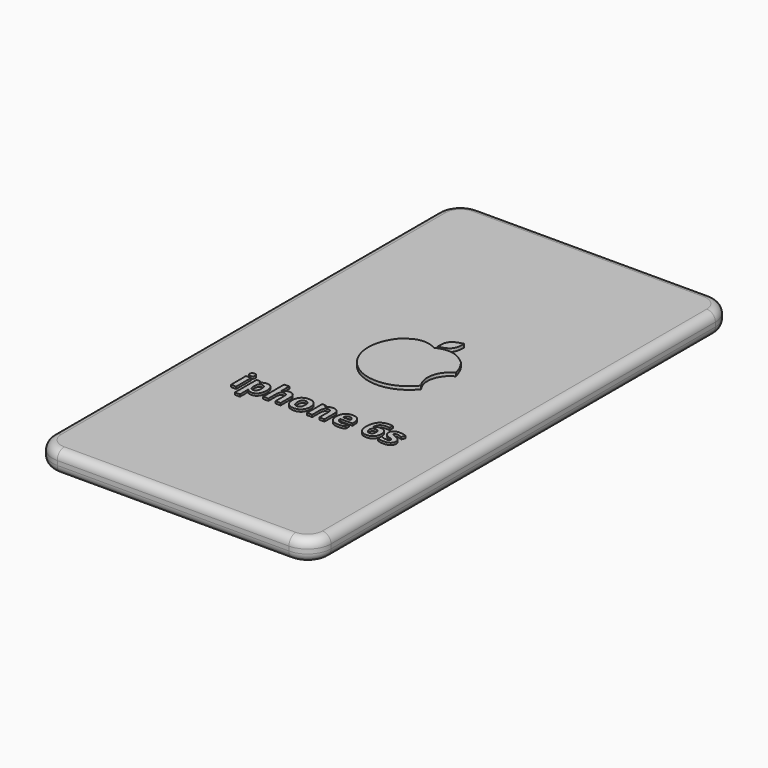
from build123d import *

# Parameters (mm, degrees)
F0_W         = 129.3353596702
F0_H         = 244.9735552073
F1_DEPTH     = 10
F3_W         = 97.1785942093
F3_H         = 200.6838843226
F3_R         = 8.9904805896
F4_DEPTH     = 1
F5_R         = 10.8639610307
F6_R         = 4
F7_TEXT_SIZE = 15.9748014994
F8_DEPTH     = 1
F10_DEPTH    = 1.5
F12_DEPTH    = 1.5


# Not quite as in the source:
# - Text() gives the source's letters only with a copy of the font that has no kerning and outlines rounded to 1/6400 em; it was checked with that copy


with BuildPart() as f1:
    # F0 (on Top) → F1 (new body)
    with BuildSketch(Plane.XY):
        with Locations((-4.1642035358, 44.1017150879)):
            Rectangle(F0_W, F0_H)
    extrude(amount=-F1_DEPTH)

    # F3 (on face) → F4 (cut)
    with BuildSketch(Plane(origin=(0, 0, -10), x_dir=(1, 0, 0), z_dir=(0, 0, -1))):
        with Locations((-4.1642035358, -38.0352623761)):
            Rectangle(F3_W, F3_H)
        with Locations((-11.1623336561, -151.3912901282)):
            Circle(F3_R)
        with BuildLine():
            ThreePointArc((-19.1459041089, 70.0142735839), (-20.1459041089, 69.0142735839), (-19.1459041089, 68.0142735839))
            Line((-19.1459041089, 68.0142735839), (0, 68.0142735839))
            ThreePointArc((0, 68.0142735839), (1, 69.0142735839), (0, 70.0142735839))
            Line((0, 70.0142735839), (-19.1459041089, 70.0142735839))
        make_face()
    extrude(amount=-F4_DEPTH, mode=Mode.SUBTRACT)

    # F5
    f5_edges = [f1.edges().sort_by_distance(p)[0] for p in [
        (-68.831883, -78.385063, -5),
        (60.503476, -78.385063, -5),
        (60.503476, 166.588493, -5),
        (-68.831883, 166.588493, -5),
    ]]
    fillet(f5_edges, radius=F5_R)

    # F6
    f6_edges = [f1.edges().sort_by_distance(p)[0] for p in [
        (-68.831883, 44.101715, 0),
        (-68.831883, 44.101715, -10),
    ]]
    fillet(f6_edges, radius=F6_R)

    # F7 (on face) → F8 (join)
    with BuildSketch(Plane.XY):
        with Locations((-41.2190929055, 0)):
            Text('iphone 6s', F7_TEXT_SIZE, font='Open Sans', font_style=FontStyle.BOLD, text_align=(TextAlign.LEFT, TextAlign.BOTTOM))
    extrude(amount=F8_DEPTH)

    # F9 (on face) → F10 (join)
    with BuildSketch(Plane.XY):
        with BuildLine():
            ThreePointArc((18.4249591586, 57.5522020899), (17.0914527335, 61.4244331789), (14.9548430037, 64.9183295505))
            add(Edge.make_bspline(
                [(0, 67.9376721382), (5.5657275952, 70.4293549061), (9.7979530466, 69.5266458432), (14.9548430037, 64.9183295505)],
                knots=[0, 0, 0, 0, 15.2565972264, 15.2565972264, 15.2565972264, 15.2565972264], degree=3))
            add(Edge.make_bspline(
                [(-14.4558428767, 65.5373054827), (-10.4473052964, 69.114478059), (-6.2707234706, 71.194827387), (0, 67.9376721382)],
                knots=[0, 0, 0, 0, 14.6537760784, 14.6537760784, 14.6537760784, 14.6537760784], degree=3))
            ThreePointArc((-14.4558428767, 65.5373054827), (-11.8718601153, 38.6756810521), (14.9324799988, 41.7983697979))
            ThreePointArc((14.9324799988, 41.7983697979), (12.9779361507, 50.4957154596), (18.4249591586, 57.5522020899))
        make_face()
    extrude(amount=F10_DEPTH)

    # F11 (on face) → F12 (join, through all)
    with BuildSketch(Plane.XY):
        with BuildLine():
            add(Edge.make_bspline(
                [(0.3618631251, 69.4593280554), (0.4521099299, 73.5039700232), (0.6456735187, 76.0559048342), (6.6407031295, 77.1566130805)],
                knots=[0, 0, 0, 0, 9.9333795134, 9.9333795134, 9.9333795134, 9.9333795134], degree=3))
            add(Edge.make_bspline(
                [(0.3618631251, 69.4593280554), (4.3059005966, 70.3603505615), (6.7669106221, 71.062680824), (6.6407031295, 77.1566130805)],
                knots=[0, 0, 0, 0, 9.9333795134, 9.9333795134, 9.9333795134, 9.9333795134], degree=3))
        make_face()
    extrude(amount=F12_DEPTH)


solid = f1.part
